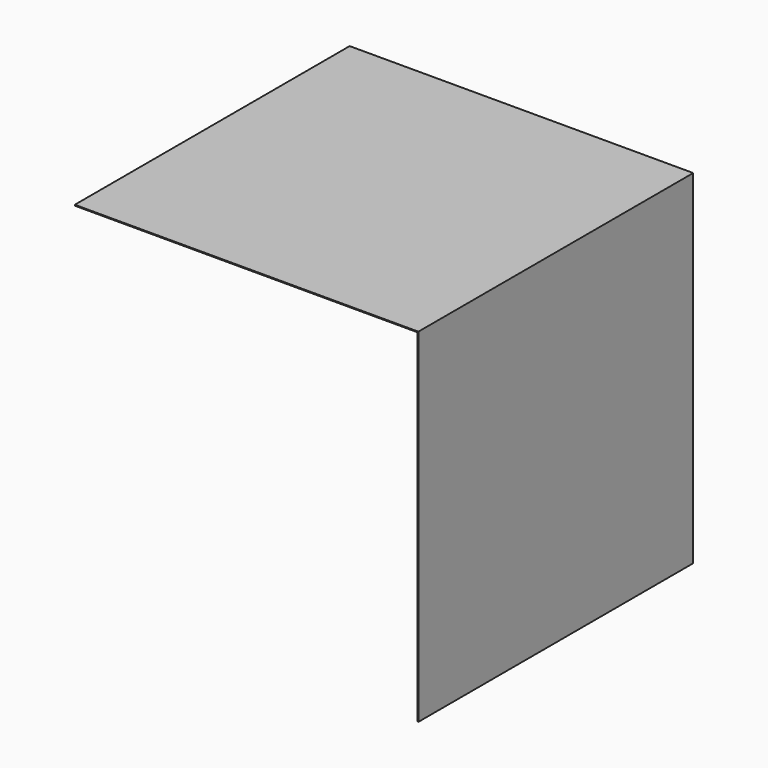
from build123d import *

# Parameters (mm, degrees)
F1_DEPTH = 25.4
F3_DEPTH = 0.127
F4_DEPTH = 50.8


with BuildPart() as f1:
    # F0 (on Front) → F1 (new body)
    with BuildSketch(Plane.XZ):
        Polygon((-0.127, 0), (0, 0), (0, 50.8), (-50.8, 50.8), (-50.8, 50.673), (-0.127, 50.673), align=None)
    extrude(amount=F1_DEPTH)

    # F0 (on Front) → F4 (join)
    with BuildSketch(Plane.XZ):
        Polygon((-0.127, 0), (0, 0), (0, 50.8), (-50.8, 50.8), (-50.8, 50.673), (-0.127, 50.673), align=None)
    extrude(amount=F4_DEPTH)


with BuildPart() as f3:
    # F2 (on face) → F3 (new body)
    with BuildSketch(Plane.XZ.offset(25.4)):
        Polygon((-4.9765948776, 50.673), (-5.1562, 50.673), (-0.127, 45.6438), (-0.127, 45.8234051224), align=None)
    extrude(amount=F3_DEPTH)


solid = Compound([f1.part, f3.part])
